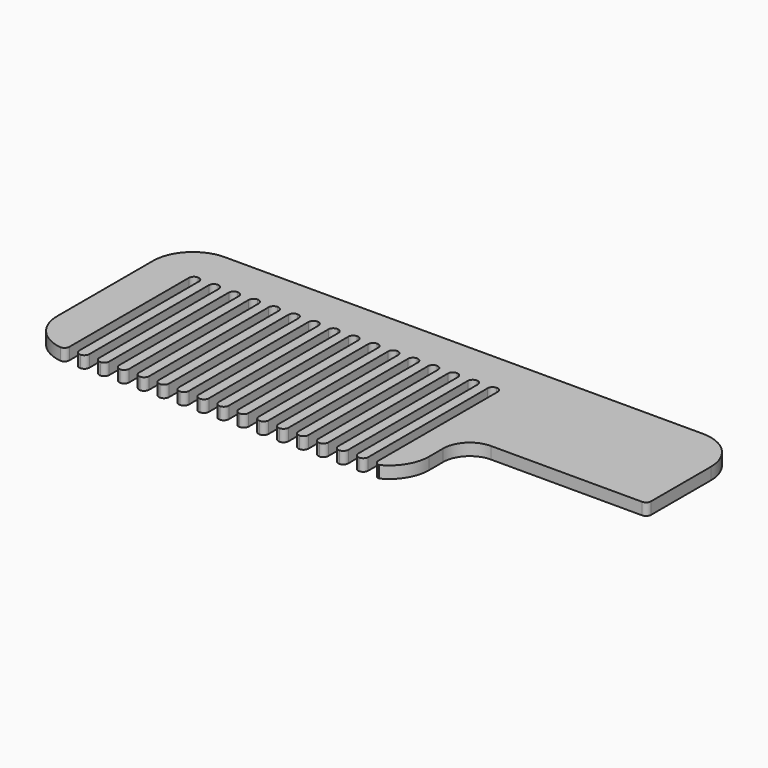
from build123d import *

# Parameters (mm, degrees)
F1_W        = 2.5
F1_H        = 40
F1_W_2      = 4.1666666667
F1_H_2      = 20
F3_DEPTH    = 3
F4_R        = 1.24999
F5_T1_DEPTH = 53
F5_T3_DEPTH = 52.6078433818
F5_T5_DEPTH = 47.4390445504
F6_R        = 6.6666666667


# Not quite as in the source:
# - a fillet or chamfer that OpenCascade refuses, or shapes differently, is made with other operations: its cross-section is extruded or revolved along the edge and cut away or added
# - a fillet or chamfer is up to 0.001 mm smaller than in the source, because OpenCascade refuses the exact size


with BuildPart() as f3:
    # F1 (on Top) → F3 (new body)
    with BuildSketch(Plane.XY):
        with Locations((38.75, 20)):
            Rectangle(F1_W, F1_H)
        with Locations((28.75, 20)):
            Rectangle(F1_W, F1_H)
        with Locations((23.75, 20)):
            Rectangle(F1_W, F1_H)
        Polygon((0, 50), (0, 0), (10, 0), (10, 40), (12.5, 40), (15, 40), (17.5, 40), (20, 40), (22.5, 40), (25, 40), (27.5, 40), (30, 40), (32.5, 40), (35, 40), (37.5, 40), (40, 40), (42.5, 40), (45, 40), (47.5, 40), (50, 40), (52.5, 40), (55, 40), (57.5, 40), (60, 40), (62.5, 40), (65, 40), (67.5, 40), (70, 40), (72.5, 40), (75, 40), (77.5, 40), (80, 40), (82.5, 40), (85, 40), (87.5, 40), (90, 40), (90, 20), (94.1666666667, 20), (140, 20), (140, 50), align=None)
        with Locations((18.75, 20)):
            Rectangle(F1_W, F1_H)
        with Locations((73.75, 20)):
            Rectangle(F1_W, F1_H)
        with Locations((13.75, 20)):
            Rectangle(F1_W, F1_H)
        with Locations((53.75, 20)):
            Rectangle(F1_W, F1_H)
        with Locations((43.75, 20)):
            Rectangle(F1_W, F1_H)
        with Locations((48.75, 20)):
            Rectangle(F1_W, F1_H)
        Polygon((90, 0), (90, 20), (90, 40), (87.5, 40), (87.5, 0), align=None)
        with Locations((68.75, 20)):
            Rectangle(F1_W, F1_H)
        with Locations((58.75, 20)):
            Rectangle(F1_W, F1_H)
        with Locations((78.75, 20)):
            Rectangle(F1_W, F1_H)
        with Locations((63.75, 20)):
            Rectangle(F1_W, F1_H)
        with Locations((83.75, 20)):
            Rectangle(F1_W, F1_H)
        with Locations((33.75, 20)):
            Rectangle(F1_W, F1_H)
        with Locations((92.0833333333, 10)):
            Rectangle(F1_W_2, F1_H_2)
    extrude(amount=F3_DEPTH)

    # F4 (radius 1.25 in the source; OpenCascade refuses exactly that, so slightly less here)
    f4_edges = [f3.edges().sort_by_distance(p)[0] for p in [
        (10, 0, 1.5),
        (12.5, 0, 1.5),
        (15, 0, 1.5),
        (17.5, 0, 1.5),
        (20, 0, 1.5),
        (22.5, 0, 1.5),
        (25, 0, 1.5),
        (27.5, 0, 1.5),
        (30, 0, 1.5),
        (32.5, 0, 1.5),
        (35, 0, 1.5),
        (37.5, 0, 1.5),
        (40, 0, 1.5),
        (42.5, 0, 1.5),
        (45, 0, 1.5),
        (47.5, 0, 1.5),
        (50, 0, 1.5),
        (52.5, 0, 1.5),
        (55, 0, 1.5),
        (57.5, 0, 1.5),
        (62.5, 0, 1.5),
        (60, 0, 1.5),
        (65, 0, 1.5),
        (67.5, 0, 1.5),
        (70, 0, 1.5),
        (72.5, 0, 1.5),
        (75, 0, 1.5),
        (77.5, 0, 1.5),
        (80, 0, 1.5),
        (82.5, 0, 1.5),
        (85, 0, 1.5),
        (87.5, 0, 1.5),
        (10, 40, 1.5),
        (15, 40, 1.5),
        (20, 40, 1.5),
        (25, 40, 1.5),
        (30, 40, 1.5),
        (35, 40, 1.5),
        (40, 40, 1.5),
        (45, 40, 1.5),
        (50, 40, 1.5),
        (85, 40, 1.5),
        (80, 40, 1.5),
        (75, 40, 1.5),
        (70, 40, 1.5),
        (65, 40, 1.5),
        (60, 40, 1.5),
        (55, 40, 1.5),
        (87.5, 40, 1.5),
        (82.5, 40, 1.5),
        (77.5, 40, 1.5),
        (72.5, 40, 1.5),
        (67.5, 40, 1.5),
        (62.5, 40, 1.5),
        (57.5, 40, 1.5),
        (52.5, 40, 1.5),
        (47.5, 40, 1.5),
        (42.5, 40, 1.5),
        (37.5, 40, 1.5),
        (32.5, 40, 1.5),
        (27.5, 40, 1.5),
        (22.5, 40, 1.5),
        (12.5, 40, 1.5),
        (17.5, 40, 1.5),
        (140, 20, 1.5),
    ]]
    fillet(f4_edges, radius=F4_R)

    # F5: fillet of radius 10 on 4 edges, made by hand

    # F5_s2 → F5_t1 (cut)
    with BuildSketch(Plane.XY.offset(-25)):
        with BuildLine():
            ThreePointArc((0, 40), (2.9289321881, 47.0710678119), (10, 50))
            Line((10, 50), (10, 50.2))
            Line((10, 50.2), (-0.2, 50.2))
            Line((-0.2, 50.2), (-0.2, 40))
            Line((-0.2, 40), (0, 40))
        make_face()
        with BuildLine():
            ThreePointArc((130, 50), (137.0710678119, 47.0710678119), (140, 40))
            Line((140, 40), (140.2, 40))
            Line((140.2, 40), (140.2, 50.2))
            Line((140.2, 50.2), (130, 50.2))
            Line((130, 50.2), (130, 50))
        make_face()
    extrude(amount=F5_T1_DEPTH, mode=Mode.SUBTRACT)

    # F5_s4 → F5_t3 (cut)
    with BuildSketch(Plane.XY.offset(-24.8039216909)):
        with BuildLine():
            ThreePointArc((8.75001, 0), (2.5000033333, 3.3071866191), (0, 9.9215686764))
            Line((0, 9.9215686764), (-0.2, 9.9215686764))
            Line((-0.2, 9.9215686764), (-0.2, 0))
            Line((-0.2, 0), (0, -0.2))
            ThreePointArc((0, -0.2), (4.375005, -0.2), (8.7250102, -0.1984313735))
            Line((8.7250102, -0.1984313735), (8.75001, 0))
        make_face()
    extrude(amount=F5_T3_DEPTH, mode=Mode.SUBTRACT)

    # F5_s6 → F5_t5 (cut)
    with BuildSketch(Plane.XY.offset(-22.2195222752)):
        with BuildLine():
            ThreePointArc((94.1666666667, 8.8878089101), (92.7057893773, 3.6836391076), (88.74999, 0))
            Line((88.74999, 0), (88.8416564667, -0.1777561782))
            ThreePointArc((88.8416564667, -0.1777561782), (91.4583283333, -0.2), (94.1666666667, -0.2))
            Line((94.1666666667, -0.2), (94.3666666667, 0))
            Line((94.3666666667, 0), (94.3666666667, 8.8878089101))
            Line((94.3666666667, 8.8878089101), (94.1666666667, 8.8878089101))
        make_face()
    extrude(amount=F5_T5_DEPTH, mode=Mode.SUBTRACT)

    # F6
    f6_edges = [f3.edges().sort_by_distance(p)[0] for p in [
        (94.166667, 20, 1.5),
    ]]
    fillet(f6_edges, radius=F6_R)


solid = f3.part
